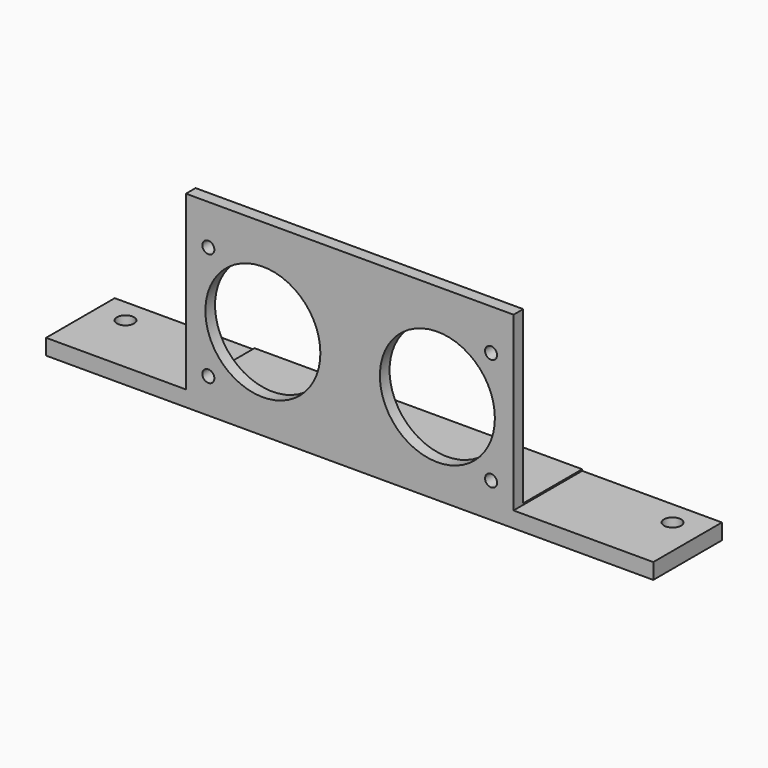
from build123d import *

# Parameters (mm, degrees)
F1_DEPTH = 2.54
F2_W     = 89.8525
F2_H     = 1.7887626846
F3_DEPTH = 50.8
F4_R     = 8.509
F4_R_2   = 0.889
F4_W     = 48.4873057247
F4_H     = 25.5061189608
F5_DEPTH = 25.4


# Not quite as in the source:
# - a feature names something its author has since deleted; it is built from what else it names


with BuildPart() as f1:
    # F0 (on Top) → F1 (new body)
    with BuildSketch(Plane.XY):
        with BuildLine():
            Line((46.9198958446, -15.3550693233), (-42.9326041554, -15.3550693233))
            Line((-42.9326041554, -15.3550693233), (-42.9326041554, -18.9255226487))
            Line((-42.9326041554, -18.9255226487), (-39.7576041554, -18.9255226487))
            ThreePointArc((-39.7576041554, -18.9255226487), (-38.4876041554, -17.6555226487), (-37.2176041554, -18.9255226487))
            Line((-37.2176041554, -18.9255226487), (41.2048958446, -18.9255226487))
            ThreePointArc((41.2048958446, -18.9255226487), (42.4748958446, -17.6555226487), (43.7448958446, -18.9255226487))
            Line((43.7448958446, -18.9255226487), (46.9198958446, -18.9255226487))
            Line((46.9198958446, -18.9255226487), (46.9198958446, -15.3550693233))
        make_face()
        with BuildLine():
            Line((-39.7576041554, -18.9255226487), (-42.9326041554, -18.9255226487))
            Line((-42.9326041554, -18.9255226487), (-42.9326041554, -28.0550693233))
            Line((-42.9326041554, -28.0550693233), (46.9198958446, -28.0550693233))
            Line((46.9198958446, -28.0550693233), (46.9198958446, -18.9255226487))
            Line((46.9198958446, -18.9255226487), (43.7448958446, -18.9255226487))
            ThreePointArc((43.7448958446, -18.9255226487), (42.4748958446, -20.1955226487), (41.2048958446, -18.9255226487))
            Line((41.2048958446, -18.9255226487), (-37.2176041554, -18.9255226487))
            ThreePointArc((-37.2176041554, -18.9255226487), (-38.4876041554, -20.1955226487), (-39.7576041554, -18.9255226487))
        make_face()
    extrude(amount=F1_DEPTH)

    # F2 (on face) → F3 (join)
    with BuildSketch(Plane.XY.offset(2.54)):
        with Locations((1.9936458446, -27.160687981)):
            Rectangle(F2_W, F2_H)
    extrude(amount=F3_DEPTH)

    # F4 (on face) → F5 (cut)
    with BuildSketch(Plane.XZ.offset(28.0550693233)):
        with Locations((-10.8520889408, 13.5200908117)):
            Circle(F4_R)
        with Locations((14.9718186097, 13.4496116212)):
            Circle(F4_R)
        with Locations((-18.9169041554, 21.9057271107)):
            Circle(F4_R_2)
        with Locations((-18.9169041554, 5.1380908117)):
            Circle(F4_R_2)
        with Locations((22.9168958446, 5.1380908117)):
            Circle(F4_R_2)
        with Locations((22.9168958446, 21.7611324307)):
            Circle(F4_R_2)
        Polygon((46.9198958446, 53.34), (26.2442958446, 53.34), (26.2442958446, 27.8338810392), (26.2442958446, 2.3277620785), (46.9198958446, 2.3277620785), align=None)
        Polygon((-22.2430098802, 53.34), (-42.9326041554, 53.34), (-42.9326041554, 2.3277620785), (-22.2430098802, 2.3277620785), (-22.2430098802, 27.8338810392), align=None)
        with Locations((2.0006429822, 40.5869405196)):
            Rectangle(F4_W, F4_H)
    extrude(amount=-F5_DEPTH, mode=Mode.SUBTRACT)


solid = f1.part
